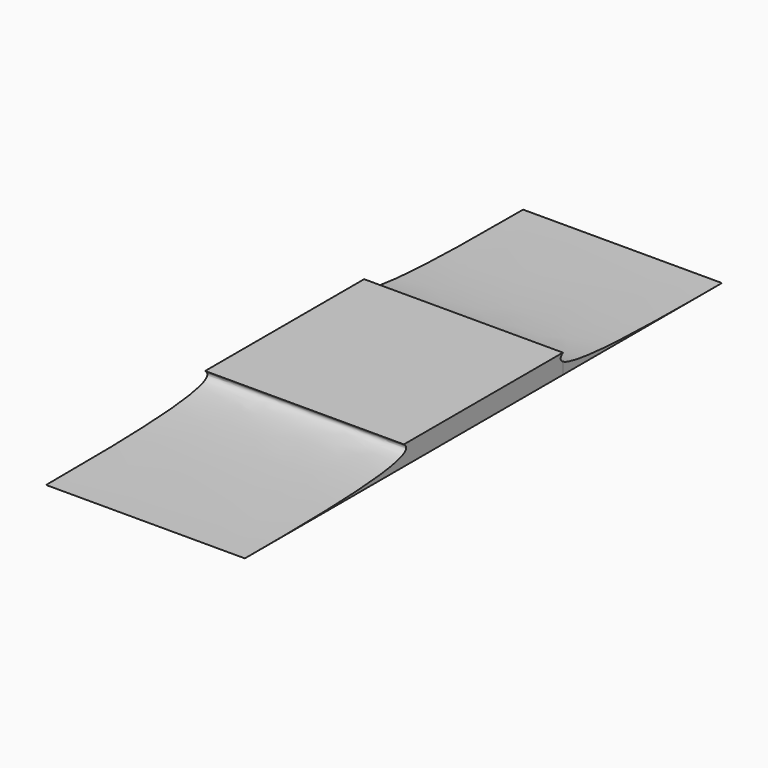
from build123d import *

# Parameters (mm, degrees)
F0_W     = 101.5999945464
F0_H     = 101.6
F1_DEPTH = 10
F2_W     = 88.9
F2_H     = 88.9
F3_DEPTH = 7.5
F4_W     = 88.9
F4_H     = 88.9
F4_H_2   = 12.7
F5_DEPTH = 3.3274
F7_DEPTH = 103.632


# Not quite as in the source:
# - ends of sketch curves that miss each other by under 0.0002 mm in the source are joined


with BuildPart() as f1:
    # F0 (on Top) → F1 (new body)
    with BuildSketch(Plane.XY):
        Polygon((-50.7999972732, 152.4), (-50.7999972732, 50.8), (50.7999972732, 50.8), (50.8000027268, 152.4), align=None)
        Rectangle(F0_W, F0_H)
        with Locations((0, -101.6)):
            Rectangle(F0_W, F0_H)
    extrude(amount=F1_DEPTH)

    # F2 (on face) → F3 (cut)
    with BuildSketch(Plane(origin=(0, 0, 0), x_dir=(1, 0, 0), z_dir=(0, 0, -1))):
        Rectangle(F2_W, F2_H)
    extrude(amount=-F3_DEPTH, mode=Mode.SUBTRACT)

    # F4 (on face) → F5 (cut)
    with BuildSketch(Plane(origin=(0, 0, 0), x_dir=(1, 0, 0), z_dir=(0, 0, -1))):
        Rectangle(F4_W, F4_H)
        with Locations((0, 50.8)):
            Rectangle(F4_W, F4_H_2)
        with Locations((0, -50.8)):
            Rectangle(F4_W, F4_H_2)
    extrude(amount=-F5_DEPTH, mode=Mode.SUBTRACT)

    # F6 (on face) → F7 (cut)
    with BuildSketch(Plane(origin=(-50.7999972732, 0, 0), x_dir=(0, -1, 0), z_dir=(-1, 0, 0))):
        with BuildLine():
            Line((-152.4, 10), (-152.4, 0))
            add(Edge.make_bspline(
                [(-152.4, 0), (-112.5093102455, 0), (-37.972824313, 0), (-50.8, 10)],
                knots=[0, 0, 0, 0, 102.0909398527, 102.0909398527, 102.0909398527, 102.0909398527], degree=3))
            Line((-50.8, 10), (-152.4, 10))
        make_face()
        with BuildLine():
            add(Edge.make_bspline(
                [(152.4, 0), (112.5093102455, 0), (37.972824313, 0), (50.8, 10)],
                knots=[0, 0, 0, 0, 102.0909398527, 102.0909398527, 102.0909398527, 102.0909398527], degree=3))
            Line((152.4, 0), (152.4, 10))
            Line((152.4, 10), (50.8, 10))
        make_face()
    extrude(amount=-F7_DEPTH, mode=Mode.SUBTRACT)


solid = f1.part
